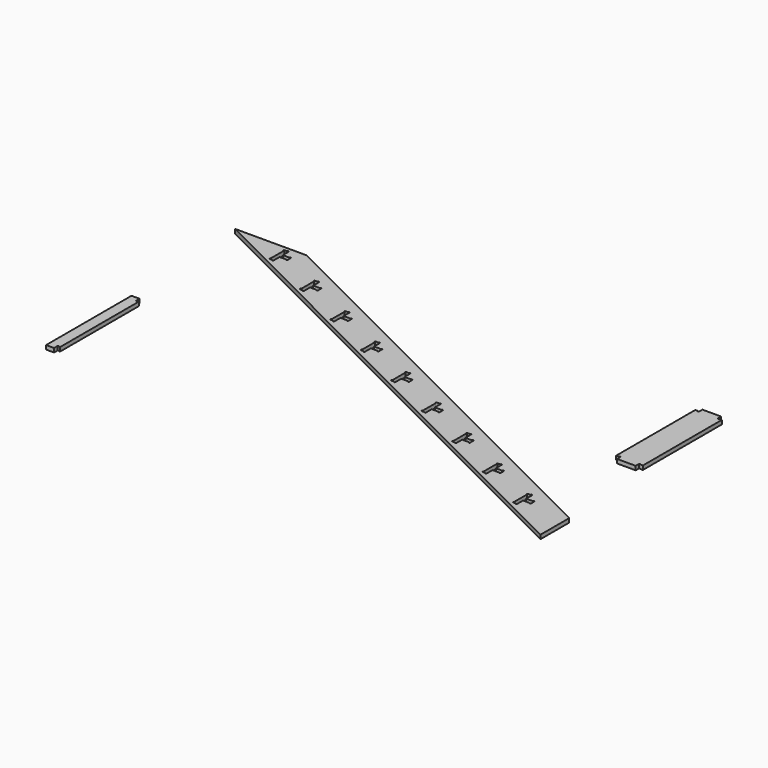
from build123d import *

# Parameters (mm, degrees)
F2_DEPTH = 19.05


# Not quite as in the source:
# - a variable given as a bare number and used for a length is read in inches; the dataset says mm whatever the document's units were
# - a feature names something its author has since deleted; it is built from what else it names


with BuildPart() as f2:
    # F1 (on Top) → F2 (new body)
    with BuildSketch(Plane.XY):
        Polygon((-1208.8109687159, 605.79), (1215.39, -606.310484358), (1215.39, -435.9221044725), (-868.034208945, 605.79), align=None)
        with BuildLine():
            ThreePointArc((974.09, -385.1221044725), (970.915, -381.9471044725), (974.09, -378.7721044725))
            Line((974.09, -378.7721044725), (986.79, -378.7721044725))
            ThreePointArc((986.79, -378.7721044725), (989.965, -375.5971044725), (993.14, -378.7721044725))
            Line((993.14, -378.7721044725), (993.14, -413.6971044725))
            Line((993.14, -413.6971044725), (1024.89, -413.6971044725))
            ThreePointArc((1024.89, -413.6971044725), (1028.065, -410.5221044725), (1031.24, -413.6971044725))
            Line((1031.24, -413.6971044725), (1031.24, -432.7471044725))
            ThreePointArc((1031.24, -432.7471044725), (1028.065, -435.9221044725), (1024.89, -432.7471044725))
            Line((1024.89, -432.7471044725), (993.14, -432.7471044725))
            Line((993.14, -432.7471044725), (993.14, -467.6721044725))
            ThreePointArc((993.14, -467.6721044725), (989.965, -470.8471044725), (986.79, -467.6721044725))
            Line((986.79, -467.6721044725), (974.09, -467.6721044725))
            ThreePointArc((974.09, -467.6721044725), (970.915, -464.4971044725), (974.09, -461.3221044725))
            Line((974.09, -461.3221044725), (974.09, -385.1221044725))
        make_face(mode=Mode.SUBTRACT)
        with BuildLine():
            ThreePointArc((491.49, -143.8221044725), (488.315, -140.6471044725), (491.49, -137.4721044725))
            Line((491.49, -137.4721044725), (504.19, -137.4721044725))
            ThreePointArc((504.19, -137.4721044725), (507.365, -134.2971044725), (510.54, -137.4721044725))
            Line((510.54, -137.4721044725), (510.54, -172.3971044725))
            Line((510.54, -172.3971044725), (542.29, -172.3971044725))
            ThreePointArc((542.29, -172.3971044725), (545.465, -169.2221044725), (548.64, -172.3971044725))
            Line((548.64, -172.3971044725), (548.64, -191.4471044725))
            ThreePointArc((548.64, -191.4471044725), (545.465, -194.6221044725), (542.29, -191.4471044725))
            Line((542.29, -191.4471044725), (510.54, -191.4471044725))
            Line((510.54, -191.4471044725), (510.54, -226.3721044725))
            ThreePointArc((510.54, -226.3721044725), (507.365, -229.5471044725), (504.19, -226.3721044725))
            Line((504.19, -226.3721044725), (491.49, -226.3721044725))
            ThreePointArc((491.49, -226.3721044725), (488.315, -223.1971044725), (491.49, -220.0221044725))
            Line((491.49, -220.0221044725), (491.49, -143.8221044725))
        make_face(mode=Mode.SUBTRACT)
        with BuildLine():
            ThreePointArc((250.19, -23.1721044725), (247.015, -19.9971044725), (250.19, -16.8221044725))
            Line((250.19, -16.8221044725), (262.89, -16.8221044725))
            ThreePointArc((262.89, -16.8221044725), (266.065, -13.6471044725), (269.24, -16.8221044725))
            Line((269.24, -16.8221044725), (269.24, -51.7471044725))
            Line((269.24, -51.7471044725), (300.99, -51.7471044725))
            ThreePointArc((300.99, -51.7471044725), (304.165, -48.5721044725), (307.34, -51.7471044725))
            Line((307.34, -51.7471044725), (307.34, -70.7971044725))
            ThreePointArc((307.34, -70.7971044725), (304.165, -73.9721044725), (300.99, -70.7971044725))
            Line((300.99, -70.7971044725), (269.24, -70.7971044725))
            Line((269.24, -70.7971044725), (269.24, -105.7221044725))
            ThreePointArc((269.24, -105.7221044725), (266.065, -108.8971044725), (262.89, -105.7221044725))
            Line((262.89, -105.7221044725), (250.19, -105.7221044725))
            ThreePointArc((250.19, -105.7221044725), (247.015, -102.5471044725), (250.19, -99.3721044725))
            Line((250.19, -99.3721044725), (250.19, -23.1721044725))
        make_face(mode=Mode.SUBTRACT)
        with BuildLine():
            ThreePointArc((732.79, -264.4721044725), (729.615, -261.2971044725), (732.79, -258.1221044725))
            Line((732.79, -258.1221044725), (745.49, -258.1221044725))
            ThreePointArc((745.49, -258.1221044725), (748.665, -254.9471044725), (751.84, -258.1221044725))
            Line((751.84, -258.1221044725), (751.84, -293.0471044725))
            Line((751.84, -293.0471044725), (783.59, -293.0471044725))
            ThreePointArc((783.59, -293.0471044725), (786.765, -289.8721044725), (789.94, -293.0471044725))
            Line((789.94, -293.0471044725), (789.94, -312.0971044725))
            ThreePointArc((789.94, -312.0971044725), (786.765, -315.2721044725), (783.59, -312.0971044725))
            Line((783.59, -312.0971044725), (751.84, -312.0971044725))
            Line((751.84, -312.0971044725), (751.84, -347.0221044725))
            ThreePointArc((751.84, -347.0221044725), (748.665, -350.1971044725), (745.49, -347.0221044725))
            Line((745.49, -347.0221044725), (732.79, -347.0221044725))
            ThreePointArc((732.79, -347.0221044725), (729.615, -343.8471044725), (732.79, -340.6721044725))
            Line((732.79, -340.6721044725), (732.79, -264.4721044725))
        make_face(mode=Mode.SUBTRACT)
        with BuildLine():
            ThreePointArc((-473.71, 338.7778955275), (-476.885, 341.9528955275), (-473.71, 345.1278955275))
            Line((-473.71, 345.1278955275), (-461.01, 345.1278955275))
            ThreePointArc((-461.01, 345.1278955275), (-457.835, 348.3028955275), (-454.66, 345.1278955275))
            Line((-454.66, 345.1278955275), (-454.66, 310.2028955275))
            Line((-454.66, 310.2028955275), (-422.91, 310.2028955275))
            ThreePointArc((-422.91, 310.2028955275), (-419.735, 313.3778955275), (-416.56, 310.2028955275))
            Line((-416.56, 310.2028955275), (-416.56, 291.1528955275))
            ThreePointArc((-416.56, 291.1528955275), (-419.735, 287.9778955275), (-422.91, 291.1528955275))
            Line((-422.91, 291.1528955275), (-454.66, 291.1528955275))
            Line((-454.66, 291.1528955275), (-454.66, 256.2278955275))
            ThreePointArc((-454.66, 256.2278955275), (-457.835, 253.0528955275), (-461.01, 256.2278955275))
            Line((-461.01, 256.2278955275), (-473.71, 256.2278955275))
            ThreePointArc((-473.71, 256.2278955275), (-476.885, 259.4028955275), (-473.71, 262.5778955275))
            Line((-473.71, 262.5778955275), (-473.71, 338.7778955275))
        make_face(mode=Mode.SUBTRACT)
        with BuildLine():
            ThreePointArc((-232.41, 218.1278955275), (-235.585, 221.3028955275), (-232.41, 224.4778955275))
            Line((-232.41, 224.4778955275), (-219.71, 224.4778955275))
            ThreePointArc((-219.71, 224.4778955275), (-216.535, 227.6528955275), (-213.36, 224.4778955275))
            Line((-213.36, 224.4778955275), (-213.36, 189.5528955275))
            Line((-213.36, 189.5528955275), (-181.61, 189.5528955275))
            ThreePointArc((-181.61, 189.5528955275), (-178.435, 192.7278955275), (-175.26, 189.5528955275))
            Line((-175.26, 189.5528955275), (-175.26, 170.5028955275))
            ThreePointArc((-175.26, 170.5028955275), (-178.435, 167.3278955275), (-181.61, 170.5028955275))
            Line((-181.61, 170.5028955275), (-213.36, 170.5028955275))
            Line((-213.36, 170.5028955275), (-213.36, 135.5778955275))
            ThreePointArc((-213.36, 135.5778955275), (-216.535, 132.4028955275), (-219.71, 135.5778955275))
            Line((-219.71, 135.5778955275), (-232.41, 135.5778955275))
            ThreePointArc((-232.41, 135.5778955275), (-235.585, 138.7528955275), (-232.41, 141.9278955275))
            Line((-232.41, 141.9278955275), (-232.41, 218.1278955275))
        make_face(mode=Mode.SUBTRACT)
        with BuildLine():
            ThreePointArc((-715.01, 459.4278955275), (-718.185, 462.6028955275), (-715.01, 465.7778955275))
            Line((-715.01, 465.7778955275), (-702.31, 465.7778955275))
            ThreePointArc((-702.31, 465.7778955275), (-699.135, 468.9528955275), (-695.96, 465.7778955275))
            Line((-695.96, 465.7778955275), (-695.96, 430.8528955275))
            Line((-695.96, 430.8528955275), (-664.21, 430.8528955275))
            ThreePointArc((-664.21, 430.8528955275), (-661.035, 434.0278955275), (-657.86, 430.8528955275))
            Line((-657.86, 430.8528955275), (-657.86, 411.8028955275))
            ThreePointArc((-657.86, 411.8028955275), (-661.035, 408.6278955275), (-664.21, 411.8028955275))
            Line((-664.21, 411.8028955275), (-695.96, 411.8028955275))
            Line((-695.96, 411.8028955275), (-695.96, 376.8778955275))
            ThreePointArc((-695.96, 376.8778955275), (-699.135, 373.7028955275), (-702.31, 376.8778955275))
            Line((-702.31, 376.8778955275), (-715.01, 376.8778955275))
            ThreePointArc((-715.01, 376.8778955275), (-718.185, 380.0528955275), (-715.01, 383.2278955275))
            Line((-715.01, 383.2278955275), (-715.01, 459.4278955275))
        make_face(mode=Mode.SUBTRACT)
        with BuildLine():
            ThreePointArc((-956.31, 580.0778955275), (-959.485, 583.2528955275), (-956.31, 586.4278955275))
            Line((-956.31, 586.4278955275), (-943.61, 586.4278955275))
            ThreePointArc((-943.61, 586.4278955275), (-940.435, 589.6028955275), (-937.26, 586.4278955275))
            Line((-937.26, 586.4278955275), (-937.26, 551.5028955275))
            Line((-937.26, 551.5028955275), (-905.51, 551.5028955275))
            ThreePointArc((-905.51, 551.5028955275), (-902.335, 554.6778955275), (-899.16, 551.5028955275))
            Line((-899.16, 551.5028955275), (-899.16, 532.4528955275))
            ThreePointArc((-899.16, 532.4528955275), (-902.335, 529.2778955275), (-905.51, 532.4528955275))
            Line((-905.51, 532.4528955275), (-937.26, 532.4528955275))
            Line((-937.26, 532.4528955275), (-937.26, 497.5278955275))
            ThreePointArc((-937.26, 497.5278955275), (-940.435, 494.3528955275), (-943.61, 497.5278955275))
            Line((-943.61, 497.5278955275), (-956.31, 497.5278955275))
            ThreePointArc((-956.31, 497.5278955275), (-959.485, 500.7028955275), (-956.31, 503.8778955275))
            Line((-956.31, 503.8778955275), (-956.31, 580.0778955275))
        make_face(mode=Mode.SUBTRACT)
        with BuildLine():
            ThreePointArc((8.89, 97.4778955275), (5.715, 100.6528955275), (8.89, 103.8278955275))
            Line((8.89, 103.8278955275), (21.59, 103.8278955275))
            ThreePointArc((21.59, 103.8278955275), (24.765, 107.0028955275), (27.94, 103.8278955275))
            Line((27.94, 103.8278955275), (27.94, 68.9028955275))
            Line((27.94, 68.9028955275), (59.69, 68.9028955275))
            ThreePointArc((59.69, 68.9028955275), (62.865, 72.0778955275), (66.04, 68.9028955275))
            Line((66.04, 68.9028955275), (66.04, 49.8528955275))
            ThreePointArc((66.04, 49.8528955275), (62.865, 46.6778955275), (59.69, 49.8528955275))
            Line((59.69, 49.8528955275), (27.94, 49.8528955275))
            Line((27.94, 49.8528955275), (27.94, 14.9278955275))
            ThreePointArc((27.94, 14.9278955275), (24.765, 11.7528955275), (21.59, 14.9278955275))
            Line((21.59, 14.9278955275), (8.89, 14.9278955275))
            ThreePointArc((8.89, 14.9278955275), (5.715, 18.1028955275), (8.89, 21.2778955275))
            Line((8.89, 21.2778955275), (8.89, 97.4778955275))
        make_face(mode=Mode.SUBTRACT)
    extrude(amount=F2_DEPTH)


with BuildPart() as f2b:
    # F1 (on Top) → F2, piece 2 (new body)
    with BuildSketch(Plane.XY):
        with BuildLine():
            Line((-1172.21, -54.61), (-1172.21, -562.61))
            Line((-1172.21, -562.61), (-1134.11, -562.61))
            Line((-1134.11, -562.61), (-1134.11, -543.56))
            ThreePointArc((-1134.11, -543.56), (-1130.935, -540.385), (-1127.76, -543.56))
            Line((-1127.76, -543.56), (-1121.41, -543.56))
            Line((-1121.41, -543.56), (-1121.41, -73.66))
            Line((-1121.41, -73.66), (-1127.76, -73.66))
            ThreePointArc((-1127.76, -73.66), (-1130.935, -76.835), (-1134.11, -73.66))
            Line((-1134.11, -73.66), (-1134.11, -54.61))
            Line((-1134.11, -54.61), (-1172.21, -54.61))
        make_face()
    extrude(amount=F2_DEPTH)


with BuildPart() as f2c:
    # F1 (on Top) → F2, piece 3 (new body)
    with BuildSketch(Plane.XY):
        with BuildLine():
            Line((1145.54, 554.99), (1056.64, 554.99))
            Line((1056.64, 554.99), (1056.64, 535.94))
            ThreePointArc((1056.64, 535.94), (1053.465, 532.765), (1050.29, 535.94))
            Line((1050.29, 535.94), (1037.59, 535.94))
            Line((1037.59, 535.94), (1037.59, 66.04))
            Line((1037.59, 66.04), (1050.29, 66.04))
            ThreePointArc((1050.29, 66.04), (1053.465, 69.215), (1056.64, 66.04))
            Line((1056.64, 66.04), (1056.64, 46.99))
            Line((1056.64, 46.99), (1145.54, 46.99))
            Line((1145.54, 46.99), (1145.54, 66.04))
            ThreePointArc((1145.54, 66.04), (1148.715, 69.215), (1151.89, 66.04))
            Line((1151.89, 66.04), (1164.59, 66.04))
            Line((1164.59, 66.04), (1164.59, 535.94))
            Line((1164.59, 535.94), (1151.89, 535.94))
            ThreePointArc((1151.89, 535.94), (1148.715, 532.765), (1145.54, 535.94))
            Line((1145.54, 535.94), (1145.54, 554.99))
        make_face()
    extrude(amount=F2_DEPTH)


solid = Compound([f2.part, f2b.part, f2c.part])
